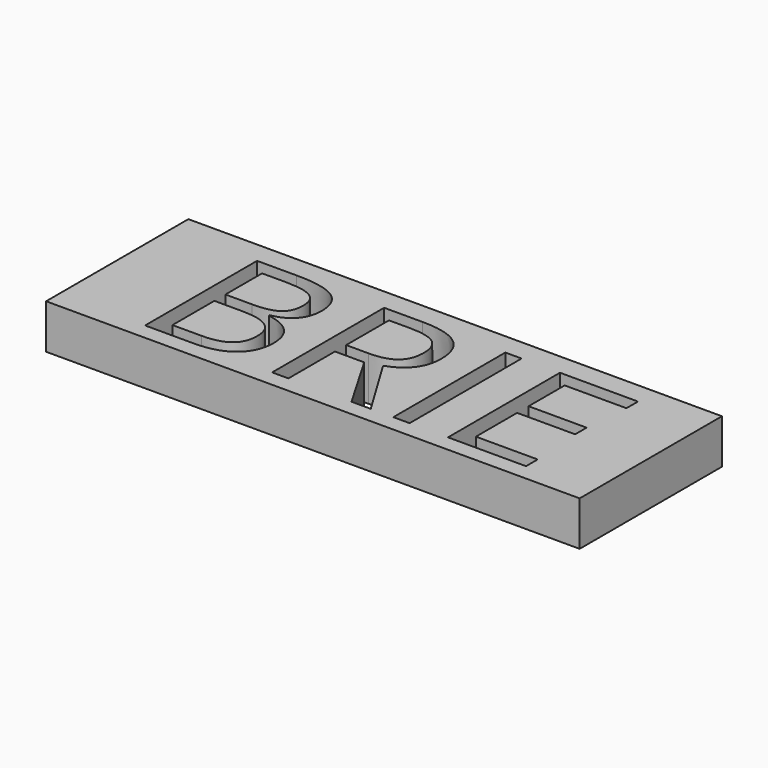
from build123d import *

# Parameters (mm, degrees)
F0_W         = 60
F0_H         = 20
F1_DEPTH     = 5
F2_TEXT_SIZE = 22.048690859
F3_DEPTH     = 5.001


# Not quite as in the source:
# - Text() gives the source's letters only with a copy of the font that has no kerning and outlines rounded to 1/6400 em; it was checked with that copy


with BuildPart() as f1:
    # F0 (on Top) → F1 (new body)
    with BuildSketch(Plane.XY):
        Rectangle(F0_W, F0_H)
    extrude(amount=F1_DEPTH)

    # F2 (on face) → F3 (cut, through all)
    with BuildSketch(Plane.XY.offset(5)):
        with Locations((-22.5, -8.1620987087)):
            Text('BRIE', F2_TEXT_SIZE, font='Open Sans', text_align=(TextAlign.LEFT, TextAlign.BOTTOM))
    extrude(amount=-F3_DEPTH, mode=Mode.SUBTRACT)


solid = f1.part
